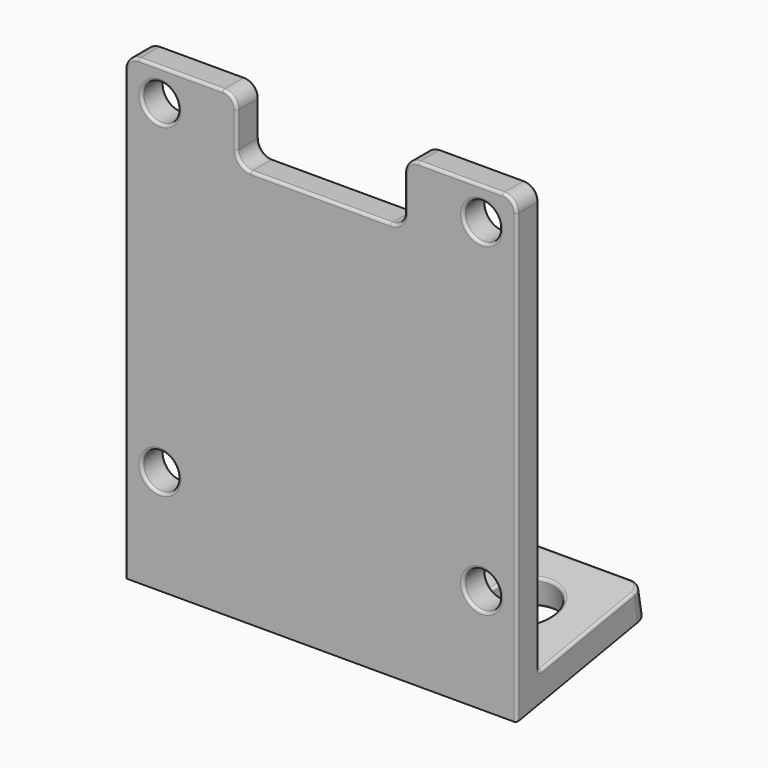
from build123d import *

# Parameters (mm, degrees)
F1_DEPTH = 14
F2_W     = 12
F2_H     = 4.5
F3_DEPTH = 25
F4_D     = 2.6
F6_D     = 4.5
F6_DEPTH = 3
F6_TIP   = 1.3519363928
F7_R     = 1
F8_R     = 0.2


# Not quite as in the source:
# - a feature names something its author has since deleted; it is built from what else it names


with BuildPart() as f1:
    # F0 (on Right) → F1 (new body, symmetric)
    with BuildSketch(Plane.YZ):
        Polygon((0, 33), (0, 0), (11.8176930361, 2.083778132), (11.4703966808, 4.053393638), (2, 2.3835071852), (2, 33), align=None)
    extrude(amount=F1_DEPTH, both=True)

    # F2 (on Front) → F3 (cut)
    with BuildSketch(Plane.XZ):
        with Locations((0, 30.75)):
            Rectangle(F2_W, F2_H)
    extrude(amount=-F3_DEPTH, mode=Mode.SUBTRACT)

    # F4 (through all)
    with Locations(Plane.XZ):
        with Locations((-11.5, 30.7), (11.5, 30.7), (11.5, 7.5), (-11.5, 7.5)):
            Hole(F4_D / 2)

    # F6
    with Locations(Plane(origin=(0, 0, 0), x_dir=(1, 0, 0), z_dir=(0, 0.1736481777, -0.984807753))):
        with Locations((-8.9999996126, -7.3), (9, -7.3)):
            Hole(F6_D / 2, depth=F6_DEPTH)
            with Locations((0, 0, -(F6_DEPTH + F6_TIP / 2))):  # 118° drill point
                Cone(0, F6_D / 2, F6_TIP, mode=Mode.SUBTRACT)

    # F7
    f7_edges = [f1.edges().sort_by_distance(p)[0] for p in [
        (-14, 1, 33),
        (14, 1, 33),
        (14, 11.644045, 3.068586),
        (-14, 11.644045, 3.068586),
        (6, 1, 33),
        (-6, 1, 33),
        (6, 1, 28.5),
        (-6, 1, 28.5),
    ]]
    fillet(f7_edges, radius=F7_R)

    # F8
    f8_edges = [f1.edges().sort_by_distance(p)[0] for p in [
        (14, 2, 17.191754),
        (13.707107, 2, 32.707107),
        (0, 2, 2.383507),
        (10, 2, 33),
        (-14, 2, 17.191754),
        (6.292893, 2, 32.707107),
        (-13.707107, 2, 32.707107),
        (6, 2, 30.75),
        (-10, 2, 33),
        (5.707107, 2, 28.792893),
        (-6.292893, 2, 32.707107),
        (0, 2, 28.5),
        (-6, 2, 30.75),
        (-5.707107, 2, 28.792893),
        (-12.8, 2, 7.5),
        (-12.8, 2, 30.7),
        (10.2, 2, 7.5),
        (10.2, 2, 30.7),
        (0, 11.470397, 4.053394),
        (-13.707107, 11.181953, 4.002533),
        (13.707107, 11.181953, 4.002533),
        (-14, 6.242794, 3.131626),
        (14, 6.242794, 3.131626),
        (-11.25, 6.8418, 3.237247),
        (6.75, 6.8418, 3.237247),
        (-10, 0, 33),
        (-6, 0, 30.75),
        (0, 0, 28.5),
        (6, 0, 30.75),
        (10, 0, 33),
        (14, 0, 16),
        (-14, 0, 16),
        (-6.292893, 0, 32.707107),
        (-13.707107, 0, 32.707107),
        (-5.707107, 0, 28.792893),
        (5.707107, 0, 28.792893),
        (13.707107, 0, 32.707107),
        (6.292893, 0, 32.707107),
        (-12.8, 0, 30.7),
        (-12.8, 0, 7.5),
        (10.2, 0, 30.7),
        (10.2, 0, 7.5),
        (-11.25, 7.189097, 1.267632),
        (6.75, 7.189097, 1.267632),
    ]]
    fillet(f8_edges, radius=F8_R)


solid = f1.part
